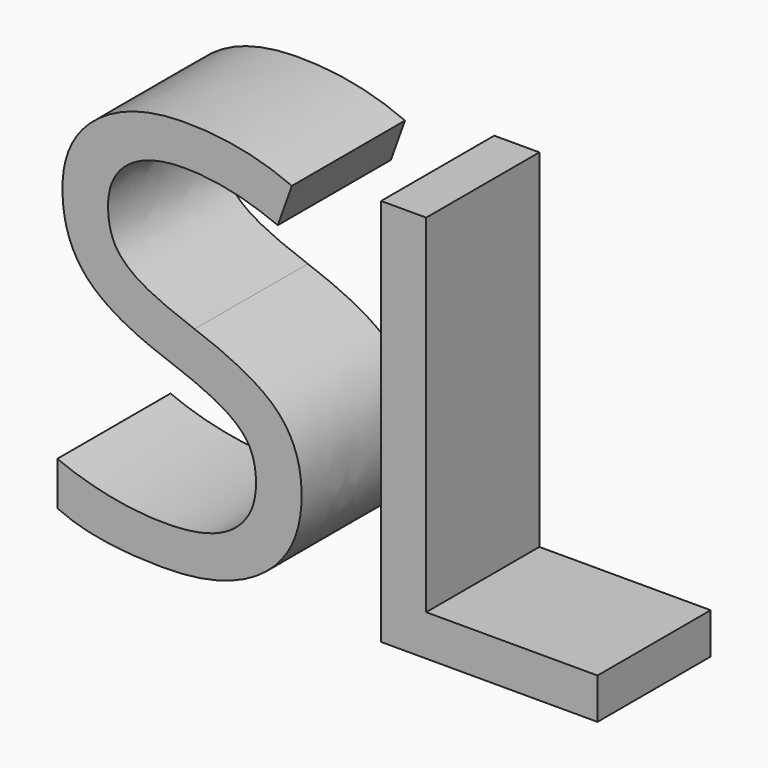
from build123d import *

# Parameters (mm, degrees)
F0_TEXT_SIZE = 97.6767546187
F1_DEPTH     = 25.4


# Not quite as in the source:
# - Text() gives the source's letters only with a copy of the font that has no kerning and outlines rounded to 1/6400 em; it was checked with that copy


with BuildPart() as f1:
    # F0 (on Front) → F1 (new body)
    with BuildSketch(Plane.XZ):
        with Locations((-53.8496188819, -39.920065552)):
            Text('SL', F0_TEXT_SIZE, font='Open Sans', text_align=(TextAlign.LEFT, TextAlign.BOTTOM))
    extrude(amount=F1_DEPTH)


solid = f1.part
